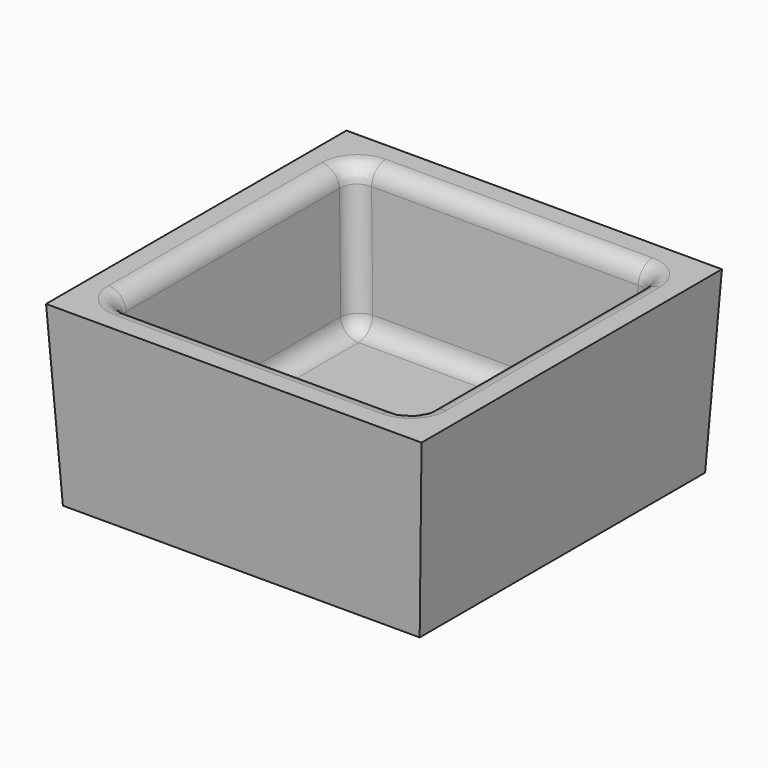
from build123d import *

# Parameters (mm, degrees)
F0_W     = 25.4
F0_H     = 25.4
F1_DEPTH = 12.7
F1_TAPER = -3
F2_T     = -2.54
F3_R     = 1.27


with BuildPart() as f1:
    # F0 (on Top) → F1 (new body)
    with BuildSketch(Plane.XY):
        Rectangle(F0_W, F0_H)
    extrude(amount=F1_DEPTH, taper=F1_TAPER)

    # F2
    f2_openings = [f1.faces().sort_by_distance(p)[0] for p in [
        (0, 0, 12.7),
    ]]
    offset(amount=F2_T, openings=f2_openings)

    # F3
    f3_edges = [f1.edges().sort_by_distance(p)[0] for p in [
        (0, -10.28963, 2.54),
        (-10.28963, 0, 2.54),
        (0, 10.28963, 2.54),
        (10.28963, 0, 2.54),
        (0, 10.822093, 12.7),
        (-10.822093, 0, 12.7),
        (0, -10.822093, 12.7),
        (10.822093, 0, 12.7),
        (-10.555862, -10.555862, 7.62),
        (10.555862, -10.555862, 7.62),
        (10.555862, 10.555862, 7.62),
        (-10.555862, 10.555862, 7.62),
    ]]
    fillet(f3_edges, radius=F3_R)


solid = f1.part
